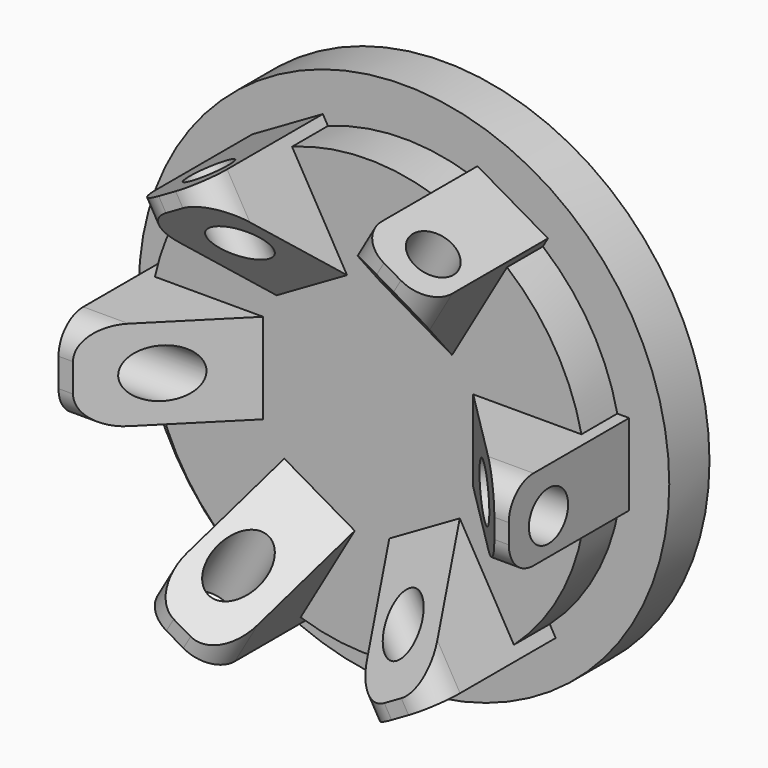
from build123d import *

# Parameters (mm, degrees)
F0_R         = 43.6202450144
F1_DEPTH     = 4.13283
F2_R         = 35.8490091113
F3_DEPTH     = 7.373
F5_DEPTH     = 28.71845
F6_T4_DEPTH  = 13.3808250539
F6_T9_DEPTH  = 1.4663911018
F7_T4_DEPTH  = 13.3808250539
F8_DEPTH     = 28.87876
F9_T4_DEPTH  = 13.3808250539
F9_T9_DEPTH  = 13.3808250539
F9_T14_DEPTH = 13.3808250539
F9_T19_DEPTH = 1.4663911018
F9_T24_DEPTH = 13.3808250539
F9_T29_DEPTH = 13.3808250539
F9_T34_DEPTH = 13.3808250539
F10_R        = 5.08
F11_R        = 4.0335860218
F12_DEPTH    = 87.80528
F14_R        = 3.8261546388
F15_DEPTH    = 90.21009
F17_R        = 3.6772087236
F18_DEPTH    = 79.11967


# Not quite as in the source:
# - a fillet or chamfer that OpenCascade refuses, or shapes differently, is made with other operations: its cross-section is extruded or revolved along the edge and cut away or added


with BuildPart() as f1:
    # F0 (on Front) → F1 (new body, symmetric)
    with BuildSketch(Plane.XZ):
        Circle(F0_R)
    extrude(amount=F1_DEPTH, both=True)

    # F2 (on face) → F3 (join)
    with BuildSketch(Plane.XZ.offset(4.13283)):
        Circle(F2_R)
    extrude(amount=F3_DEPTH)

    # F4 (on Front) → F5 (join)
    with BuildSketch(Plane.XZ):
        Polygon((-16.8635044247, 7.4236080982), (-37.0263941586, 7.4236080982), (-37.0263941586, 5.957217045), (-37.0263941586, -5.9572169557), (-37.0263941765, -7.4236080089), (-16.8635044426, -7.4236080575), (-16.863504439, -5.9572169557), (-16.8635044247, -5.224020686), (-16.8635044247, 5.2240207266), (-16.8635044247, 5.9572169964), align=None)
        Polygon((37.0263941586, 7.4236080982), (16.8635044247, 7.4236080982), (16.8635044247, -5.224020686), (16.8635044247, -5.9572169557), (37.0263941586, -5.9572169557), align=None)
        Polygon((24.9422302573, -28.3539939228), (14.8607854044, -10.8924191915), (3.9076175745, -17.2162335748), (3.2726509787, -17.5828317091), (13.3540958316, -35.0444064405), align=None)
        Polygon((-12.084163936, -35.7776019816), (-2.002719041, -18.3160272745), (-12.9558868556, -11.9922128648), (-13.5908534505, -11.6256147289), (-23.6722983455, -29.087189436), align=None)
        Polygon((-24.9422301889, 28.3539939829), (-14.8607853781, 10.8924192273), (-3.907617533, 17.2162335842), (-3.2726509363, 17.582831717), (-13.3540957472, 35.0444064727), align=None)
        Polygon((12.0841640223, 35.7776019524), (2.0027190852, 18.3160272697), (12.9558868845, 11.9922128336), (13.5908534786, 11.6256146962), (23.6722984157, 29.0871893789), align=None)
    extrude(amount=F5_DEPTH)

    # F6: chamfer of 17.78 on 1 edges, made by hand


with BuildPart() as f6_tool2:
    # F6_s3 → F6_t4 (new body)
    with BuildSketch(Plane.XY.offset(-5.9572169557)):
        with BuildLine():
            Line((-35.1463987747, -29.2213443428), (-16.3606100891, -10.4355556572))
            Line((-16.3606100891, -10.4355556572), (-16.0050100891, -10.4355556572))
            ThreePointArc((-16.0050100891, -10.4355556572), (-16.5079044319, -19.5770028286), (-16.5079044319, -28.71845))
            Line((-16.5079044319, -28.71845), (-16.8635044319, -29.07405))
            ThreePointArc((-16.8635044319, -29.07405), (-26.0049516033, -29.07405), (-35.1463987747, -29.5769443428))
            Line((-35.1463987747, -29.5769443428), (-35.1463987747, -29.2213443428))
        make_face()
    extrude(amount=F6_T4_DEPTH)

    split(bisect_by=Plane.XZ.offset(11.50583), keep=Keep.TOP)


with BuildPart() as f1_1:
    add(f1.part)

    # F6_t1: cut F6_tool2
    add(f6_tool2.part, mode=Mode.SUBTRACT)


with BuildPart() as f6_tool7:
    # F6_s8 → F6_t9 (new body)
    with BuildSketch(Plane.XY.offset(-7.4236080575)):
        with BuildLine():
            Line((-35.1463987854, -29.2213443428), (-16.3606100998, -10.4355556572))
            Line((-16.3606100998, -10.4355556572), (-16.0050100998, -10.4355556572))
            ThreePointArc((-16.0050100998, -10.4355556572), (-16.5079044426, -19.5770028286), (-16.5079044426, -28.71845))
            Line((-16.5079044426, -28.71845), (-16.8635044426, -29.07405))
            ThreePointArc((-16.8635044426, -29.07405), (-26.004951614, -29.07405), (-35.1463987854, -29.5769443428))
            Line((-35.1463987854, -29.5769443428), (-35.1463987854, -29.2213443428))
        make_face()
    extrude(amount=F6_T9_DEPTH)

    split(bisect_by=Plane.XZ.offset(11.50583), keep=Keep.TOP)


with BuildPart() as f1_2:
    add(f1_1.part)

    # F6_t6: cut F6_tool7
    add(f6_tool7.part, mode=Mode.SUBTRACT)

    # F7: chamfer of 17.78 on 1 edges, made by hand


with BuildPart() as f7_tool2:
    # F7_s3 → F7_t4 (new body)
    with BuildSketch(Plane.XY.offset(7.4236080982)):
        with BuildLine():
            Line((35.1463987675, -29.2213443428), (16.3606100819, -10.4355556572))
            Line((16.3606100819, -10.4355556572), (16.0050100819, -10.4355556572))
            ThreePointArc((16.0050100819, -10.4355556572), (16.5079044247, -19.5770028286), (16.5079044247, -28.71845))
            Line((16.5079044247, -28.71845), (16.8635044247, -29.07405))
            ThreePointArc((16.8635044247, -29.07405), (26.0049515961, -29.07405), (35.1463987675, -29.5769443428))
            Line((35.1463987675, -29.5769443428), (35.1463987675, -29.2213443428))
        make_face()
    extrude(amount=-F7_T4_DEPTH)

    split(bisect_by=Plane.XZ.offset(11.50583), keep=Keep.TOP)


with BuildPart() as f1_3:
    add(f1_2.part)

    # F7_t1: cut F7_tool2
    add(f7_tool2.part, mode=Mode.SUBTRACT)

    # F4 (on Front) → F8 (join)
    with BuildSketch(Plane.XZ):
        Polygon((-16.8635044247, 7.4236080982), (-37.0263941586, 7.4236080982), (-37.0263941586, 5.957217045), (-37.0263941586, -5.9572169557), (-37.0263941765, -7.4236080089), (-16.8635044426, -7.4236080575), (-16.863504439, -5.9572169557), (-16.8635044247, -5.224020686), (-16.8635044247, 5.2240207266), (-16.8635044247, 5.9572169964), align=None)
        Polygon((37.0263941586, 7.4236080982), (16.8635044247, 7.4236080982), (16.8635044247, -5.224020686), (16.8635044247, -5.9572169557), (37.0263941586, -5.9572169557), align=None)
        Polygon((24.9422302573, -28.3539939228), (14.8607854044, -10.8924191915), (3.9076175745, -17.2162335748), (3.2726509787, -17.5828317091), (13.3540958316, -35.0444064405), align=None)
        Polygon((-12.084163936, -35.7776019816), (-2.002719041, -18.3160272745), (-12.9558868556, -11.9922128648), (-13.5908534505, -11.6256147289), (-23.6722983455, -29.087189436), align=None)
        Polygon((-24.9422301889, 28.3539939829), (-14.8607853781, 10.8924192273), (-3.907617533, 17.2162335842), (-3.2726509363, 17.582831717), (-13.3540957472, 35.0444064727), align=None)
        Polygon((12.0841640223, 35.7776019524), (2.0027190852, 18.3160272697), (12.9558868845, 11.9922128336), (13.5908534786, 11.6256146962), (23.6722984157, 29.0871893789), align=None)
    extrude(amount=F8_DEPTH)

    # F9: chamfer of 17.78 on 7 edges, made by hand


with BuildPart() as f9_tool2:
    # F9_s3 → F9_t4 (new body)
    with BuildSketch(Plane(origin=(-6.4290331859, 0, 3.7118040749), x_dir=(0, 1, 0), z_dir=(0.8660254018, 0, -0.5000000035))):
        with BuildLine():
            Line((-10.5958656572, 16.3606100819), (-29.3816543428, 35.1463987675))
            Line((-29.3816543428, 35.1463987675), (-29.7372543428, 35.1463987675))
            ThreePointArc((-29.7372543428, 35.1463987675), (-29.23436, 26.0049515961), (-29.23436, 16.8635044247))
            Line((-29.23436, 16.8635044247), (-28.87876, 16.5079044247))
            ThreePointArc((-28.87876, 16.5079044247), (-19.7373128286, 16.5079044247), (-10.5958656572, 16.0050100819))
            Line((-10.5958656572, 16.0050100819), (-10.5958656572, 16.3606100819))
        make_face()
    extrude(amount=F9_T4_DEPTH)

    split(bisect_by=Plane.XZ.offset(11.50583), keep=Keep.TOP)


with BuildPart() as f1_4:
    add(f1_3.part)

    # F9_t1: cut F9_tool2
    add(f9_tool2.part, mode=Mode.SUBTRACT)


with BuildPart() as f9_tool7:
    # F9_s8 → F9_t9 (new body)
    with BuildSketch(Plane(origin=(-6.4290332127, 0, -3.7118040284), x_dir=(0, 1, 0), z_dir=(0.8660254054, 0, 0.4999999972))):
        with BuildLine():
            Line((-10.5958656572, 16.3606100819), (-29.3816543428, 35.1463987675))
            Line((-29.3816543428, 35.1463987675), (-29.7372543428, 35.1463987675))
            ThreePointArc((-29.7372543428, 35.1463987675), (-29.23436, 26.0049515961), (-29.23436, 16.8635044247))
            Line((-29.23436, 16.8635044247), (-28.87876, 16.5079044247))
            ThreePointArc((-28.87876, 16.5079044247), (-19.7373128286, 16.5079044247), (-10.5958656572, 16.0050100819))
            Line((-10.5958656572, 16.0050100819), (-10.5958656572, 16.3606100819))
        make_face()
    extrude(amount=F9_T9_DEPTH)

    split(bisect_by=Plane.XZ.offset(11.50583), keep=Keep.TOP)


with BuildPart() as f1_5:
    add(f1_4.part)

    # F9_t6: cut F9_tool7
    add(f9_tool7.part, mode=Mode.SUBTRACT)


with BuildPart() as f9_tool12:
    # F9_s13 → F9_t14 (new body)
    with BuildSketch(Plane.XY.offset(-5.9572169557)):
        with BuildLine():
            Line((-35.1463987747, -29.3816543428), (-16.3606100891, -10.5958656572))
            Line((-16.3606100891, -10.5958656572), (-16.0050100891, -10.5958656572))
            ThreePointArc((-16.0050100891, -10.5958656572), (-16.5079044319, -19.7373128286), (-16.5079044319, -28.87876))
            Line((-16.5079044319, -28.87876), (-16.8635044319, -29.23436))
            ThreePointArc((-16.8635044319, -29.23436), (-26.0049516033, -29.23436), (-35.1463987747, -29.7372543428))
            Line((-35.1463987747, -29.7372543428), (-35.1463987747, -29.3816543428))
        make_face()
    extrude(amount=F9_T14_DEPTH)

    split(bisect_by=Plane.XZ.offset(11.50583), keep=Keep.TOP)


with BuildPart() as f1_6:
    add(f1_5.part)

    # F9_t11: cut F9_tool12
    add(f9_tool12.part, mode=Mode.SUBTRACT)


with BuildPart() as f9_tool17:
    # F9_s18 → F9_t19 (new body)
    with BuildSketch(Plane.XY.offset(-7.4236080575)):
        with BuildLine():
            Line((-16.3606100998, -10.5958656572), (-35.1463987854, -29.3816543428))
            Line((-35.1463987854, -29.3816543428), (-35.1463987854, -29.7372543428))
            ThreePointArc((-35.1463987854, -29.7372543428), (-26.004951614, -29.23436), (-16.8635044426, -29.23436))
            Line((-16.8635044426, -29.23436), (-16.5079044426, -28.87876))
            ThreePointArc((-16.5079044426, -28.87876), (-16.5079044426, -19.7373128286), (-16.0050100998, -10.5958656572))
            Line((-16.0050100998, -10.5958656572), (-16.3606100998, -10.5958656572))
        make_face()
    extrude(amount=F9_T19_DEPTH)

    split(bisect_by=Plane.XZ.offset(11.50583), keep=Keep.TOP)


with BuildPart() as f1_7:
    add(f1_6.part)

    # F9_t16: cut F9_tool17
    add(f9_tool17.part, mode=Mode.SUBTRACT)


with BuildPart() as f9_tool22:
    # F9_s23 → F9_t24 (new body)
    with BuildSketch(Plane(origin=(6.4290331948, 0, -3.7118040594), x_dir=(0, 1, 0), z_dir=(-0.866025403, 0, 0.5000000014))):
        with BuildLine():
            Line((-10.5958656572, 16.3606100819), (-29.3816543428, 35.1463987675))
            Line((-29.3816543428, 35.1463987675), (-29.7372543428, 35.1463987675))
            ThreePointArc((-29.7372543428, 35.1463987675), (-29.23436, 26.0049515961), (-29.23436, 16.8635044247))
            Line((-29.23436, 16.8635044247), (-28.87876, 16.5079044247))
            ThreePointArc((-28.87876, 16.5079044247), (-19.7373128286, 16.5079044247), (-10.5958656572, 16.0050100819))
            Line((-10.5958656572, 16.0050100819), (-10.5958656572, 16.3606100819))
        make_face()
    extrude(amount=F9_T24_DEPTH)

    split(bisect_by=Plane.XZ.offset(11.50583), keep=Keep.TOP)


with BuildPart() as f1_8:
    add(f1_7.part)

    # F9_t21: cut F9_tool22
    add(f9_tool22.part, mode=Mode.SUBTRACT)


with BuildPart() as f9_tool27:
    # F9_s28 → F9_t29 (new body)
    with BuildSketch(Plane(origin=(6.4290332037, 0, 3.7118040439), x_dir=(0, 1, 0), z_dir=(-0.8660254042, 0, -0.4999999993))):
        with BuildLine():
            Line((-10.5958656572, 16.3606100819), (-29.3816543428, 35.1463987675))
            Line((-29.3816543428, 35.1463987675), (-29.7372543428, 35.1463987675))
            ThreePointArc((-29.7372543428, 35.1463987675), (-29.23436, 26.0049515961), (-29.23436, 16.8635044247))
            Line((-29.23436, 16.8635044247), (-28.87876, 16.5079044247))
            ThreePointArc((-28.87876, 16.5079044247), (-19.7373128286, 16.5079044247), (-10.5958656572, 16.0050100819))
            Line((-10.5958656572, 16.0050100819), (-10.5958656572, 16.3606100819))
        make_face()
    extrude(amount=F9_T29_DEPTH)

    split(bisect_by=Plane.XZ.offset(11.50583), keep=Keep.TOP)


with BuildPart() as f1_9:
    add(f1_8.part)

    # F9_t26: cut F9_tool27
    add(f9_tool27.part, mode=Mode.SUBTRACT)


with BuildPart() as f9_tool32:
    # F9_s33 → F9_t34 (new body)
    with BuildSketch(Plane.XY.offset(7.4236080982)):
        with BuildLine():
            Line((16.3606100819, -10.5958656572), (35.1463987675, -29.3816543428))
            Line((35.1463987675, -29.3816543428), (35.1463987675, -29.7372543428))
            ThreePointArc((35.1463987675, -29.7372543428), (26.0049515961, -29.23436), (16.8635044247, -29.23436))
            Line((16.8635044247, -29.23436), (16.5079044247, -28.87876))
            ThreePointArc((16.5079044247, -28.87876), (16.5079044247, -19.7373128286), (16.0050100819, -10.5958656572))
            Line((16.0050100819, -10.5958656572), (16.3606100819, -10.5958656572))
        make_face()
    extrude(amount=-F9_T34_DEPTH)

    split(bisect_by=Plane.XZ.offset(11.50583), keep=Keep.TOP)


with BuildPart() as f1_10:
    add(f1_9.part)

    # F9_t31: cut F9_tool32
    add(f9_tool32.part, mode=Mode.SUBTRACT)

    # F10
    f10_edges = [f1_10.edges().sort_by_distance(p)[0] for p in [
        (12.758373, -28.87876, -34.012585),
        (24.346508, -28.87876, -27.322172),
        (-11.488442, -28.87876, -34.74578),
        (-23.076576, -28.87876, -28.055368),
        (-35.834949, -28.87876, -7.423608),
        (-35.834949, -28.87876, 7.423608),
        (35.834949, -28.87876, 7.423608),
        (35.834949, -28.87876, -5.957217),
        (23.076576, -28.87876, 28.055368),
        (11.488442, -28.87876, 34.74578),
        (-24.346508, -28.87876, 27.322172),
        (-12.758373, -28.87876, 34.012585),
    ]]
    fillet(f10_edges, radius=F10_R)

    # F11 (on face) → F12 (cut)
    with BuildSketch(Plane.YZ.offset(37.0263941586)):
        with Locations((-20.7159072161, 0)):
            Circle(F11_R)
    extrude(amount=-F12_DEPTH, mode=Mode.SUBTRACT)

    # F14 (on face) → F15 (cut)
    with BuildSketch(Plane(origin=(18.5131972081, 0, 32.0657978775), x_dir=(0.8660254018, 0, -0.5000000035), z_dir=(0.5000000035, 0, 0.8660254018))):
        with Locations((0, -21.2672781199)):
            Circle(F14_R)
    extrude(amount=-F15_DEPTH, mode=Mode.SUBTRACT)

    # F17 (on face) → F18 (cut)
    with BuildSketch(Plane(origin=(18.5131970535, 0, -32.0657979668), x_dir=(0.8660254042, 0, 0.4999999993), z_dir=(0.4999999993, 0, -0.8660254042))):
        with Locations((0, 21.0790149868)):
            Circle(F17_R)
    extrude(amount=-F18_DEPTH, mode=Mode.SUBTRACT)


solid = f1_10.part
